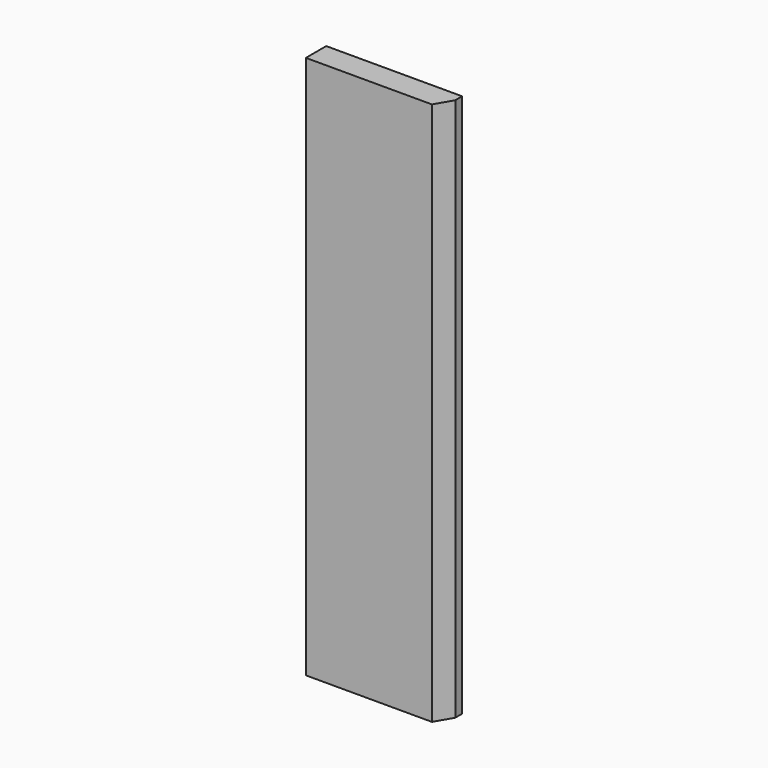
from build123d import *

# Parameters (mm, degrees)
F0_W     = 50.8
F0_H     = 203.2
F1_DEPTH = 9.525
F2_SIZE2 = 3.6661742094
F2_SIZE  = 6.35


# Not quite as in the source:
# - a length typed as a fraction of an inch, garbled in the dataset ("3 / 203.2 mm" for 3/8 in), is restored


with BuildPart() as f1:
    # F0 (on Front) → F1 (new body)
    with BuildSketch(Plane.XZ):
        with Locations((-1.7615184188, 42.1527517154)):
            Rectangle(F0_W, F0_H)
    extrude(amount=F1_DEPTH)

    # F2
    f2_edges = [f1.edges().sort_by_distance(p)[0] for p in [
        (23.638482, -9.525, 42.152752),
    ]]
    f2_side = f1.faces().sort_by_distance((23.638482, -4.7625, 42.152752))[0]
    chamfer(f2_edges, length=F2_SIZE, length2=F2_SIZE2, reference=f2_side)


solid = f1.part
